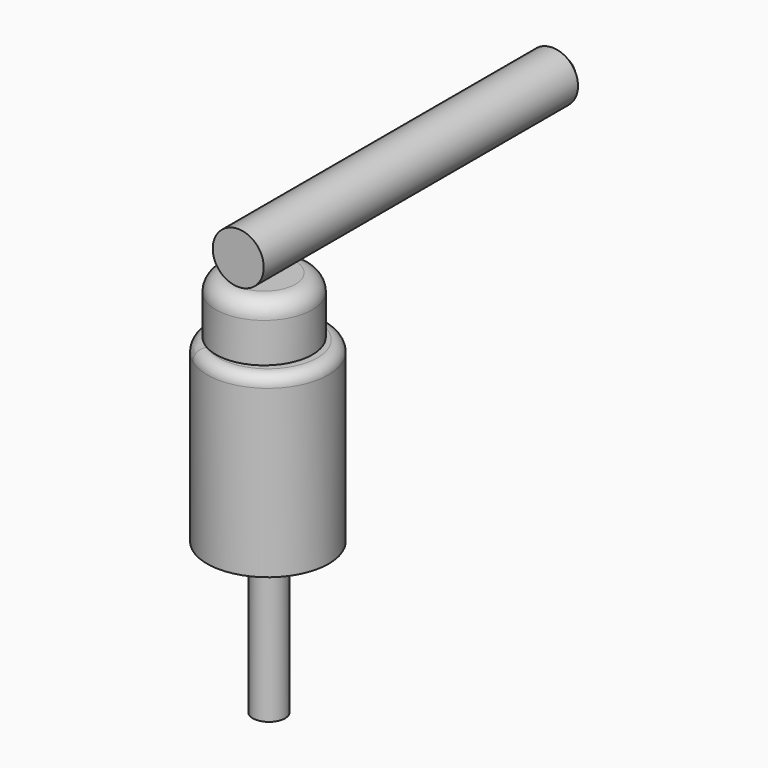
from build123d import *

# Parameters (mm, degrees)
F0_R     = 27.3395312078
F1_DEPTH = 79.83503
F2_R     = 21.6676000415
F3_DEPTH = 25.4
F6_R     = 11.4685905788
F7_DEPTH = 181.65072
F8_R     = 7.2692434599
F9_DEPTH = 67.23363
F10_R    = 5.08
F11_R    = 7.62
F12_SIZE = 5.08


with BuildPart() as f1:
    # F0 (on Top) → F1 (new body)
    with BuildSketch(Plane.XY):
        with Locations((-36.4448577166, 17.9913379252)):
            Circle(F0_R)
    extrude(amount=F1_DEPTH)

    # F2 (on face) → F3 (join)
    with BuildSketch(Plane.XY.offset(79.83503)):
        with Locations((-38.7377776206, 18.7697913498)):
            Circle(F2_R)
    extrude(amount=F3_DEPTH)

    # F8 (on face) → F9 (join)
    with BuildSketch(Plane(origin=(0, 0, 0), x_dir=(1, 0, 0), z_dir=(0, 0, -1))):
        with Locations((-35.6188900769, -17.5687633455)):
            Circle(F8_R)
    extrude(amount=F9_DEPTH)

    # F10
    f10_edges = [f1.edges().sort_by_distance(p)[0] for p in [
        (-63.784389, 17.991338, 79.83503),
    ]]
    fillet(f10_edges, radius=F10_R)

    # F11
    f11_edges = [f1.edges().sort_by_distance(p)[0] for p in [
        (-60.405378, 18.769791, 105.23503),
    ]]
    fillet(f11_edges, radius=F11_R)


with BuildPart() as f7:
    # F6 (on face) → F7 (new body)
    with BuildSketch(Plane.XZ.offset(-4.2296172571)):
        with Locations((-38.7658327818, 116.9691085815)):
            Circle(F6_R)
    extrude(amount=-F7_DEPTH)

    # F12
    f12_edges = [f7.edges().sort_by_distance(p)[0] for p in [
        (-50.234423, 185.880337, 116.969109),
    ]]
    chamfer(f12_edges, length=F12_SIZE)


solid = Compound([f1.part, f7.part])
